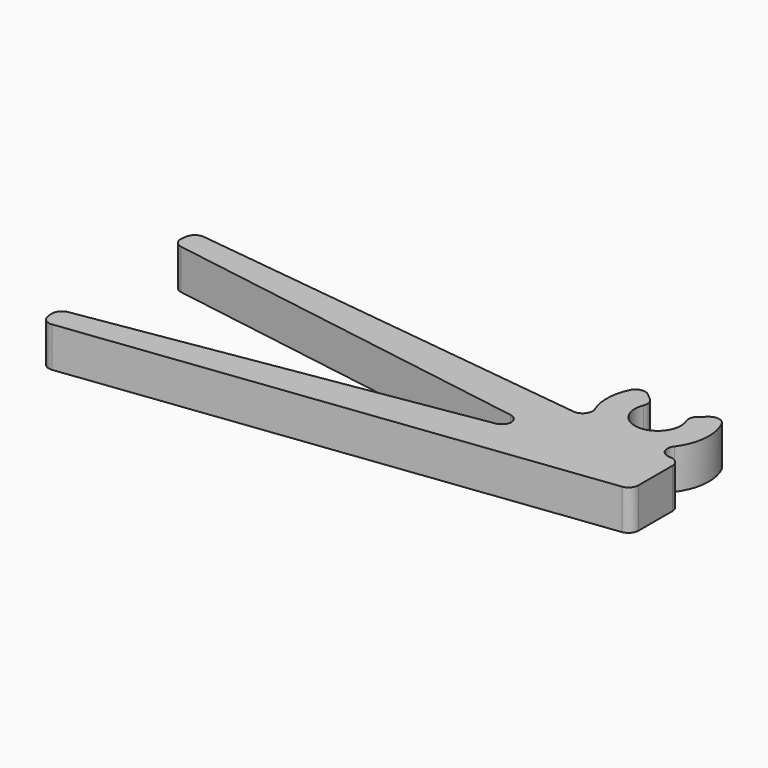
from build123d import *

# Parameters (mm, degrees)
F1_DEPTH     = 1
F2_T1_DEPTH  = 2
F2_T3_DEPTH  = 4.1120925968
F2_T5_DEPTH  = 5.1335042229
F2_T7_DEPTH  = 4.211585233
F2_T9_DEPTH  = 4.4058060179
F2_T11_DEPTH = 4.5


# Not quite as in the source:
# - a fillet or chamfer that OpenCascade refuses, or shapes differently, is made with other operations: its cross-section is extruded or revolved along the edge and cut away or added


with BuildPart() as f1:
    # F0 (on Top) → F1 (new body, symmetric)
    with BuildSketch(Plane.XY):
        with BuildLine():
            Line((-19.8, -3.608959583), (-19.6536349592, -4.8))
            Line((-19.6536349592, -4.8), (7.2, -1.5))
            Line((7.2, -1.5), (7.2, 1.5))
            Line((7.2, 1.5), (5.5036997956, 1.7084556032))
            ThreePointArc((5.5036997956, 1.7084556032), (6.7140946083, 3.4735867022), (6.15341333, 5.5391084047))
            Line((6.15341333, 5.5391084047), (5.0809511096, 4.6392057511))
            ThreePointArc((5.0809511096, 4.6392057511), (4.2, 2.75), (3.3190488904, 4.6392057511))
            Line((3.3190488904, 4.6392057511), (2.24658667, 5.5391084047))
            ThreePointArc((2.24658667, 5.5391084047), (1.6526664248, 3.7834167399), (2.4044726286, 2.089314644))
            Line((2.4044726286, 2.089314644), (-19.6536349592, 4.8))
            Line((-19.6536349592, 4.8), (-19.8, 3.608959583))
            Line((-19.8, 3.608959583), (0, 0.4))
            Line((0, 0.4), (0, -0.4))
            Line((0, -0.4), (-19.8, -3.608959583))
        make_face()
    extrude(amount=F1_DEPTH, both=True)

    # F2: fillet of radius 0.5 on 14 edges, made by hand

    # F2_s2 → F2_t1 (join)
    with BuildSketch(Plane.XY.offset(-1)):
        with BuildLine():
            ThreePointArc((-0.4200093847, -0.4680703606), (-0.1192144254, -0.2985509875), (0, 0.0254896676))
            Line((0, 0.0254896676), (0, -0.4))
            Line((0, -0.4), (-0.4200093847, -0.4680703606))
        make_face()
        with BuildLine():
            ThreePointArc((0, -0.0254896676), (-0.1192144254, 0.2985509875), (-0.4200093847, 0.4680703606))
            Line((-0.4200093847, 0.4680703606), (0, 0.4))
            Line((0, 0.4), (0, -0.0254896676))
        make_face()
        with BuildLine():
            ThreePointArc((6.2414791759, 2.3719742233), (6.1818236662, 1.8762743647), (6.5807837768, 1.5760944855))
            Line((6.5807837768, 1.5760944855), (5.5036997956, 1.7084556032))
            ThreePointArc((5.5036997956, 1.7084556032), (5.9051744273, 2.003983077), (6.2414791759, 2.3719742233))
        make_face()
        with BuildLine():
            ThreePointArc((1.3273886474, 2.2216757617), (1.7871578534, 2.4163277766), (1.8492963629, 2.9117225034))
            ThreePointArc((1.8492963629, 2.9117225034), (2.0864966132, 2.4732542504), (2.4044726286, 2.089314644))
            Line((2.4044726286, 2.089314644), (1.3273886474, 2.2216757617))
        make_face()
    extrude(amount=F2_T1_DEPTH)

    # F2_s4 → F2_t3 (cut)
    with BuildSketch(Plane.XY.offset(-2.0560462984)):
        with BuildLine():
            ThreePointArc((3.1364686576, 4.3374940957), (3.1595895158, 4.6471438712), (2.995457531, 4.9107311415))
            Line((2.995457531, 4.9107311415), (3.3190488904, 4.6392057511))
            ThreePointArc((3.3190488904, 4.6392057511), (3.2161247629, 4.4953902231), (3.1364686576, 4.3374940957))
        make_face()
        with BuildLine():
            ThreePointArc((5.404542469, 4.9107311415), (5.2404104842, 4.6471438712), (5.2635313424, 4.3374940957))
            ThreePointArc((5.2635313424, 4.3374940957), (5.1838752371, 4.4953902231), (5.0809511096, 4.6392057511))
            Line((5.0809511096, 4.6392057511), (5.404542469, 4.9107311415))
        make_face()
    extrude(amount=F2_T3_DEPTH, mode=Mode.SUBTRACT)

    # F2_s6 → F2_t5 (cut)
    with BuildSketch(Plane.XY.offset(-2.5667521115)):
        with BuildLine():
            ThreePointArc((1.9057976578, 5.0131646836), (2.2511861931, 5.283864521), (2.6770350591, 5.1779193202))
            Line((2.6770350591, 5.1779193202), (2.24658667, 5.5391084047))
            ThreePointArc((2.24658667, 5.5391084047), (2.0599733824, 5.2866456202), (1.9057976578, 5.0131646836))
        make_face()
        with BuildLine():
            ThreePointArc((6.4942023422, 5.0131646836), (6.1488138069, 5.283864521), (5.7229649409, 5.1779193202))
            Line((5.7229649409, 5.1779193202), (6.15341333, 5.5391084047))
            ThreePointArc((6.15341333, 5.5391084047), (6.3400266176, 5.2866456202), (6.4942023422, 5.0131646836))
        make_face()
    extrude(amount=F2_T5_DEPTH, mode=Mode.SUBTRACT)

    # F2_s8 → F2_t7 (cut)
    with BuildSketch(Plane.XY.offset(-2.1057926165)):
        with BuildLine():
            ThreePointArc((7.2, 1.0576829534), (7.0744948043, 1.388973825), (6.7609854337, 1.5539497938))
            Line((6.7609854337, 1.5539497938), (7.2, 1.5))
            Line((7.2, 1.5), (7.2, 1.0576829534))
        make_face()
        with BuildLine():
            ThreePointArc((6.7609854337, -1.5539497938), (7.0744948043, -1.388973825), (7.2, -1.0576829534))
            Line((7.2, -1.0576829534), (7.2, -1.5))
            Line((7.2, -1.5), (6.7609854337, -1.5539497938))
        make_face()
    extrude(amount=F2_T7_DEPTH, mode=Mode.SUBTRACT)

    # F2_s10 → F2_t9 (cut)
    with BuildSketch(Plane.XY.offset(-2.202903009)):
        with BuildLine():
            ThreePointArc((-19.3250361256, -3.5319828216), (-19.644918404, -3.7253734495), (-19.7413123507, -4.0865282835))
            Line((-19.7413123507, -4.0865282835), (-19.8, -3.608959583))
            Line((-19.8, -3.608959583), (-19.3250361256, -3.5319828216))
        make_face()
        with BuildLine():
            ThreePointArc((-19.7413123507, 4.0865282835), (-19.644918404, 3.7253734495), (-19.3250361256, 3.5319828216))
            Line((-19.3250361256, 3.5319828216), (-19.8, 3.608959583))
            Line((-19.8, 3.608959583), (-19.7413123507, 4.0865282835))
        make_face()
    extrude(amount=F2_T9_DEPTH, mode=Mode.SUBTRACT)

    # F2_s12 → F2_t11 (cut)
    with BuildSketch(Plane.XY.offset(-2.25)):
        with BuildLine():
            ThreePointArc((-19.7146203929, -4.3037331596), (-19.5261439869, -4.6367845878), (-19.1573681188, -4.7390145663))
            Line((-19.1573681188, -4.7390145663), (-19.6536349592, -4.8))
            Line((-19.6536349592, -4.8), (-19.7146203929, -4.3037331596))
        make_face()
        with BuildLine():
            ThreePointArc((-19.1573681188, 4.7390145663), (-19.5261439869, 4.6367845878), (-19.7146203929, 4.3037331596))
            Line((-19.7146203929, 4.3037331596), (-19.6536349592, 4.8))
            Line((-19.6536349592, 4.8), (-19.1573681188, 4.7390145663))
        make_face()
    extrude(amount=F2_T11_DEPTH, mode=Mode.SUBTRACT)


solid = f1.part
